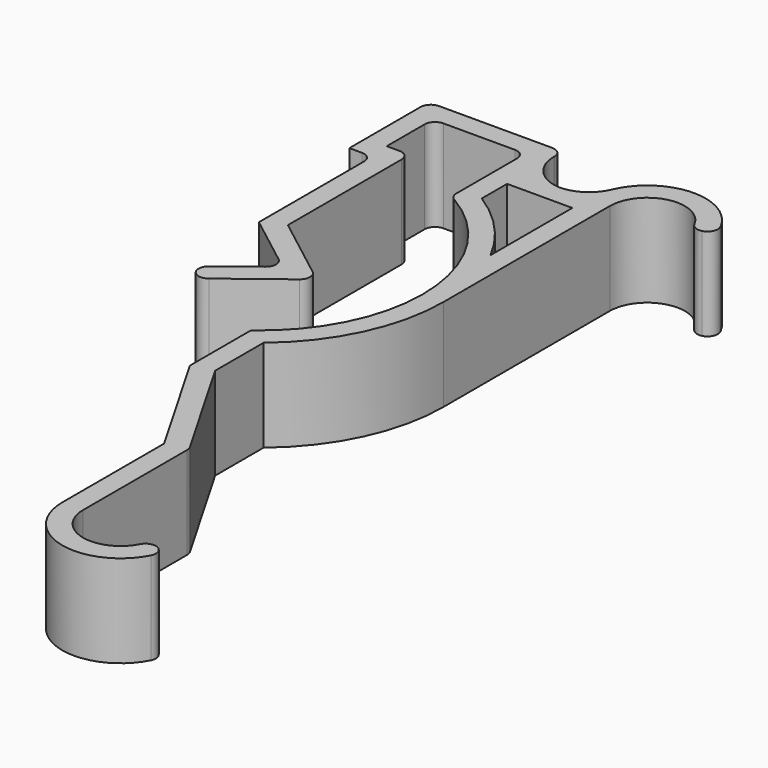
from build123d import *

# Parameters (mm, degrees)
F1_DEPTH    = 8
F2_R        = 0.89999
F3_T1_DEPTH = 8


# Not quite as in the source:
# - a fillet or chamfer that OpenCascade refuses, or shapes differently, is made with other operations: its cross-section is extruded or revolved along the edge and cut away or added
# - a fillet or chamfer is up to 0.001 mm smaller than in the source, because OpenCascade refuses the exact size
# - a feature names something its author has since deleted; it is built from what else it names


with BuildPart() as f1:
    # F0 (on Top) → F1 (new body)
    with BuildSketch(Plane.XY):
        with BuildLine():
            ThreePointArc((0, 57), (2.8257898753, 60.2221957995), (6.3892589354, 57.8411618966))
            Line((6.3892589354, 57.8411618966), (8.1279254228, 58.3070361778))
            ThreePointArc((8.1279254228, 58.3070361778), (2.5908427293, 62.0067965499), (-1.8, 57))
            Line((-1.8, 57), (-7.45, 57))
            Line((-7.45, 57), (-7.45, 61.2228588262))
            Line((-7.45, 61.2228588262), (-9.7, 61.2228588262))
            Line((-9.7, 61.2228588262), (-19.05, 61.2228588262))
            Line((-19.05, 61.2228588262), (-19.05, 52.6228588262))
            Line((-19.05, 52.6228588262), (-17.05, 52.6228588262))
            Line((-17.05, 52.6228588262), (-17.05, 40.3365361308))
            Line((-17.05, 40.3365361308), (-11.702219504, 36.2228588262))
            Line((-11.702219504, 36.2228588262), (-16.3474793695, 32.6495820066))
            Line((-16.3474793695, 32.6495820066), (-15.25, 31.2228588262))
            Line((-15.25, 31.2228588262), (-8.75, 36.2228588262))
            Line((-8.75, 36.2228588262), (-15.25, 41.2228588262))
            Line((-15.25, 41.2228588262), (-15.25, 54.4228588262))
            Line((-15.25, 54.4228588262), (-17.25, 54.4228588262))
            Line((-17.25, 54.4228588262), (-17.25, 59.4228588262))
            Line((-17.25, 59.4228588262), (-9.25, 59.4228588262))
            Line((-9.25, 59.4228588262), (-9.25, 57))
            Line((-9.25, 57), (-9.25, 51.4228588262))
            ThreePointArc((-9.25, 51.4228588262), (-3.8052690832, 46.2427536444), (-1.8, 39))
            ThreePointArc((-1.8, 39), (-3.3260618955, 32.624044706), (-7.5735026919, 27.6299564509))
            Line((-7.5735026919, 27.6299564509), (-7.5735026919, 21.0176914536))
            Line((-7.5735026919, 21.0176914536), (-1.8, 11.0176914536))
            Line((-1.8, 11.0176914536), (-1.8, 0))
            ThreePointArc((-1.8, 0), (2.5908427293, -5.0067965499), (8.1279254228, -1.3070361778))
            Line((8.1279254228, -1.3070361778), (6.3892589354, -0.8411618966))
            ThreePointArc((6.3892589354, -0.8411618966), (2.8257898753, -3.2221957995), (0, 0))
            Line((0, 0), (0, 11.5))
            Line((0, 11.5), (-5.7735026919, 21.5))
            Line((-5.7735026919, 21.5), (-5.7735026919, 26.75))
            ThreePointArc((-5.7735026919, 26.75), (-1.5156985287, 32.2288141117), (0, 39))
            Line((0, 39), (0, 57))
        make_face()
        with BuildLine():
            Line((-7.45, 55.2), (-1.8, 55.2))
            Line((-1.8, 55.2), (-1.8, 46.3441924145))
            ThreePointArc((-1.8, 46.3441924145), (-4.2171968015, 49.7784455096), (-7.45, 52.4591018057))
            Line((-7.45, 52.4591018057), (-7.45, 55.2))
        make_face(mode=Mode.SUBTRACT)
    extrude(amount=F1_DEPTH)

    # F2 (radius 0.9 in the source; OpenCascade refuses exactly that, so slightly less here)
    f2_edges = [f1.edges().sort_by_distance(p)[0] for p in [
        (8.127925, 58.307036, 4),
        (6.389259, 57.841162, 4),
        (8.127925, -1.307036, 4),
        (6.389259, -0.841162, 4),
        (-11.70222, 36.222859, 4),
        (-16.347479, 32.649582, 4),
        (-15.25, 31.222859, 4),
        (-8.75, 36.222859, 4),
        (-17.25, 59.422859, 4),
        (-15.25, 54.422859, 4),
        (-9.25, 59.422859, 4),
        (-19.05, 61.222859, 4),
        (-17.05, 52.622859, 4),
        (-9.25, 51.422859, 4),
        (0, 11.5, 4),
        (-7.45, 61.222859, 4),
    ]]
    fillet(f2_edges, radius=F2_R)

    # F3: fillet of radius 3.25 on 2 edges, made by hand

    # F3_s2 → F3_t1 (join)
    with BuildSketch(Plane.XY):
        with BuildLine():
            ThreePointArc((-4.2, 57), (-6.4980970389, 57.9519029611), (-7.45, 60.25))
            Line((-7.45, 60.25), (-7.45, 57))
            Line((-7.45, 57), (-4.2, 57))
        make_face()
        with BuildLine():
            ThreePointArc((-1.3967570543, 58.9774096386), (-2.5946788815, 57.5390574817), (-4.3872442674, 57))
            Line((-4.3872442674, 57), (-1.8, 57))
            ThreePointArc((-1.8, 57), (-1.698162443, 58.0090532384), (-1.3967570543, 58.9774096386))
        make_face()
    extrude(amount=F3_T1_DEPTH)


solid = f1.part
